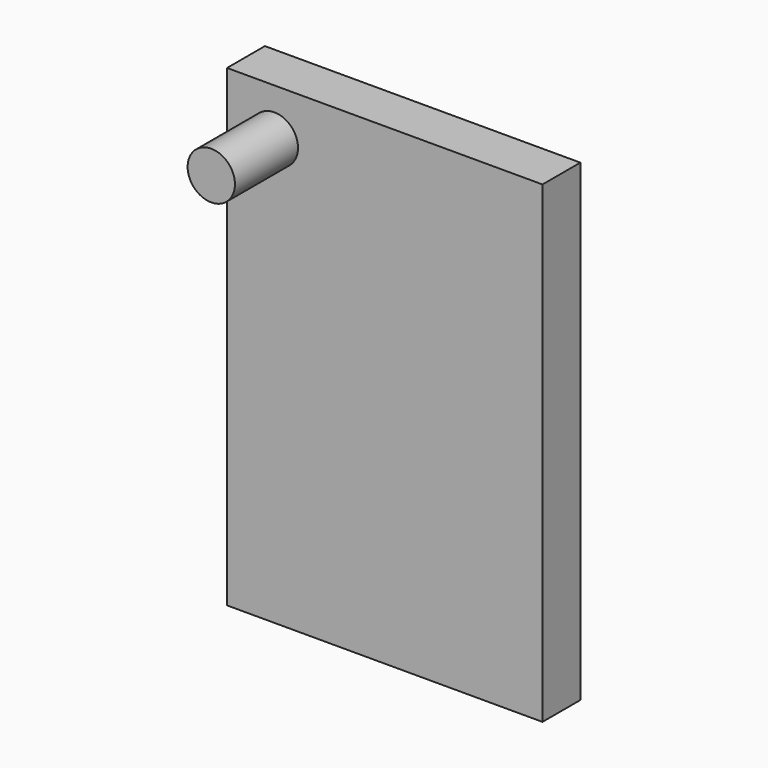
from build123d import *

# Parameters (mm, degrees)
F0_W     = 20
F0_H     = 30
F1_DEPTH = 3
F2_R     = 1.5
F3_DEPTH = 5


# Not quite as in the source:
# - a feature names something its author has since deleted; it is built from what else it names


with BuildPart() as f1:
    # F0 (on Front) → F1 (new body)
    with BuildSketch(Plane.XZ):
        with Locations((3.3097672276, -12)):
            Rectangle(F0_W, F0_H)
    extrude(amount=F1_DEPTH)

    # F2 (on face) → F3 (join)
    with BuildSketch(Plane.XZ.offset(3)):
        with Locations((-3.6902327724, 0)):
            Circle(F2_R)
    extrude(amount=F3_DEPTH)


solid = f1.part
